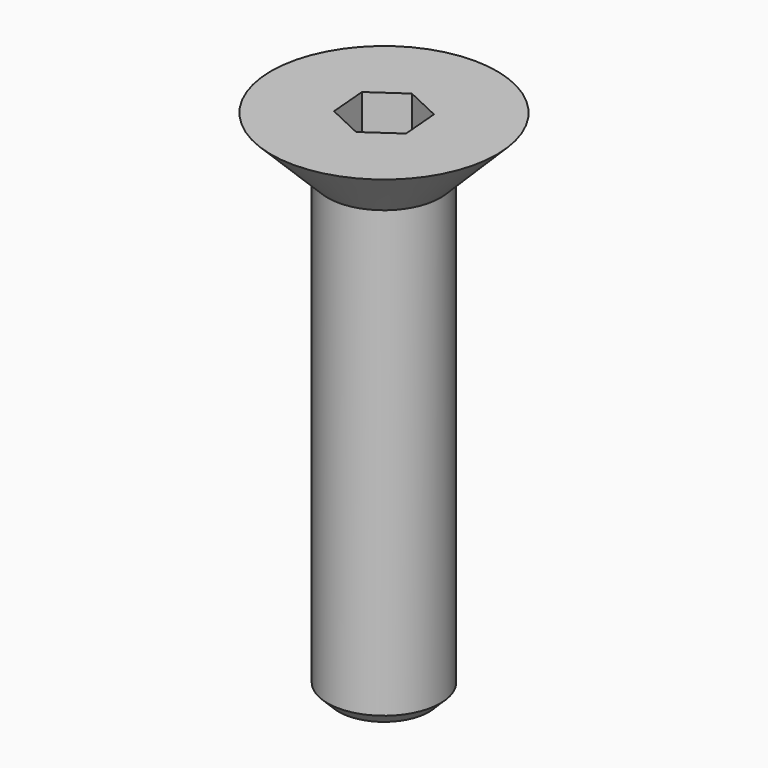
from build123d import *

# Parameters (mm, degrees)
F0_R        = 5
F1_DEPTH    = 2.7
F4_DEPTH    = 2
F2_R        = 2.5
F5_DEPTH    = 20
F6_SIZE     = 0.5
F7_S5_R     = 2.5
F7_T6_DEPTH = 9


# Not quite as in the source:
# - a fillet or chamfer that OpenCascade refuses, or shapes differently, is made with other operations: its cross-section is extruded or revolved along the edge and cut away or added
# - a feature names something its author has since deleted; it is built from what else it names


with BuildPart() as f1:
    # F0 (on Top) → F1 (new body)
    with BuildSketch(Plane.XY):
        Circle(F0_R)
    extrude(amount=F1_DEPTH)

    # F3 (on face) → F4 (cut)
    with BuildSketch(Plane.XY.offset(2.7)):
        Polygon((1.4221256636, 0.98871563), (-0.1451900209, 1.725954767), (-1.5673156845, 0.737239137), (-1.4221256636, -0.98871563), (0.1451900209, -1.725954767), (1.5673156845, -0.737239137), align=None)
    extrude(amount=-F4_DEPTH, mode=Mode.SUBTRACT)

    # F2 (on face) → F5 (join)
    with BuildSketch(Plane(origin=(0, 0, 0), x_dir=(1, 0, 0), z_dir=(0, 0, -1))):
        Circle(F2_R)
    extrude(amount=F5_DEPTH)

    # F6
    f6_edges = [f1.edges().sort_by_distance(p)[0] for p in [
        (-2.5, 0, -20),
    ]]
    chamfer(f6_edges, length=F6_SIZE)

    # F7: chamfer of 2.7 on 1 edges, made by hand


with BuildPart() as f7_tool2:
    # F7_s3 → F7_t4 (revolve)
    with BuildSketch(Plane.XZ):
        Polygon((2.3, 0), (5, 2.7), (5, 0), align=None)
    revolve(axis=Axis((0, 0, 0), (0, 0, 1)))

    # F7_s5 → F7_t6 (cut, symmetric)
    with BuildSketch(Plane.XY.offset(1.4)):
        Circle(F7_S5_R)
    extrude(amount=F7_T6_DEPTH, both=True, mode=Mode.SUBTRACT)


with BuildPart() as f1_1:
    add(f1.part)

    # F7_t1: cut F7_tool2
    add(f7_tool2.part, mode=Mode.SUBTRACT)


solid = f1_1.part
